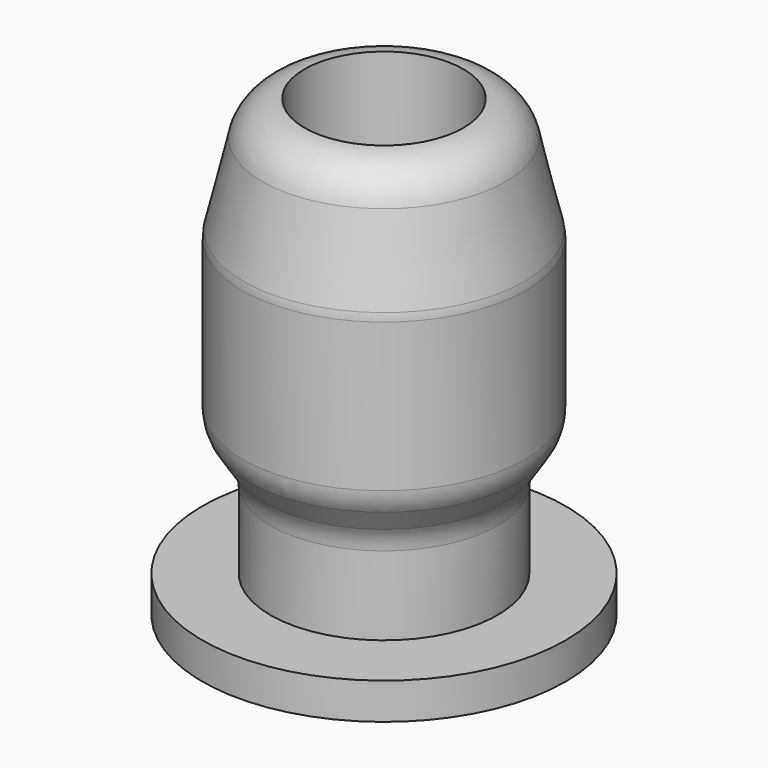
from build123d import *

# Parameters (mm, degrees)
F2_R     = 1.75
F3_DEPTH = 25


# Not quite as in the source:
# - a fillet or chamfer that OpenCascade refuses, or shapes differently, is made with other operations: its cross-section is extruded or revolved along the edge and cut away or added


with BuildPart() as f1:
    # F0 (on Front) → F1 (revolve)
    with BuildSketch(Plane.XZ):
        Polygon((-4, 0), (0, 0), (0, 10), (-2.5, 10), (-3.1176584307, 7.3764383901), (-3.1176584307, 3.7520567627), (-2.5, 2.8), (-2.5, 0.8), (-4, 0.8), align=None)
    revolve(axis=Axis((0, 0, 5), (0, 0, 1)))

    # F2 (on face) → F3 (cut)
    with BuildSketch(Plane.XY.offset(10)):
        Circle(F2_R)
    extrude(amount=-F3_DEPTH, mode=Mode.SUBTRACT)

    # F4: fillet of radius 1 on 7 edges, made by hand

    # F4_s1 → F4_t2 (revolve)
    with BuildSketch(Plane.XZ):
        with BuildLine():
            ThreePointArc((-2.4996, 2.5034415217), (-2.5408144836, 2.7879202783), (-2.6610688008, 3.0490058884))
            Line((-2.6610688008, 3.0490058884), (-2.5769756809, 3.1035623251))
            ThreePointArc((-2.5769756809, 3.1035623251), (-2.4966090641, 2.9789505293), (-2.4159068801, 2.8545564367))
            Line((-2.4159068801, 2.8545564367), (-2.39976, 2.8))
            ThreePointArc((-2.39976, 2.8), (-2.39976, 2.6517207608), (-2.39936, 2.5034415217))
            Line((-2.39936, 2.5034415217), (-2.4996, 2.5034415217))
        make_face()
    revolve(axis=Axis((0, 0, 2.8), (0, 0, 1)))

    # F4_s3 → F4_t4 (revolve, cut)
    with BuildSketch(Plane.XZ):
        with BuildLine():
            ThreePointArc((-1.7069387157, 10.0004), (-2.3289092353, 9.7839522663), (-2.6821291124, 9.2281351497))
            Line((-2.6821291124, 9.2281351497), (-2.7796481521, 9.251093809))
            ThreePointArc((-2.7796481521, 9.251093809), (-2.6883889182, 9.6369804016), (-2.5975190397, 10.0229586592))
            Line((-2.5975190397, 10.0229586592), (-2.5, 10.1001851443))
            ThreePointArc((-2.5, 10.1001851443), (-2.1034693578, 10.1001851443), (-1.7069387157, 10.1005851443))
            Line((-1.7069387157, 10.1005851443), (-1.7069387157, 10.0004))
        make_face()
    revolve(axis=Axis((0, 0, 10), (0, 0, 1)), mode=Mode.SUBTRACT)

    # F4_s5 → F4_t6 (revolve, cut)
    with BuildSketch(Plane.XZ):
        with BuildLine():
            ThreePointArc((-3.0913827866, 7.489792119), (-3.1113671869, 7.3757078111), (-3.1180584307, 7.2600798179))
            Line((-3.1180584307, 7.2600798179), (-3.2182984307, 7.2600798179))
            ThreePointArc((-3.2182984307, 7.2600798179), (-3.2178984307, 7.318259104), (-3.2178984307, 7.3764383901))
            Line((-3.2178984307, 7.3764383901), (-3.2152308663, 7.3994096202))
            ThreePointArc((-3.2152308663, 7.3994096202), (-3.2018983666, 7.4560406522), (-3.1889552222, 7.5127633491))
            Line((-3.1889552222, 7.5127633491), (-3.0913827866, 7.489792119))
        make_face()
    revolve(axis=Axis((0, 0, 7.3764383901), (0, 0, 1)), mode=Mode.SUBTRACT)

    # F4_s7 → F4_t8 (revolve, cut)
    with BuildSketch(Plane.XZ):
        with BuildLine():
            ThreePointArc((-3.1180584307, 4.048615241), (-3.0768439472, 3.7641364844), (-2.9565896299, 3.5030508742))
            Line((-2.9565896299, 3.5030508742), (-3.0406827498, 3.4484944376))
            ThreePointArc((-3.0406827498, 3.4484944376), (-3.1210493667, 3.5731062334), (-3.2017515506, 3.697500326))
            Line((-3.2017515506, 3.697500326), (-3.2178984307, 3.7520567627))
            ThreePointArc((-3.2178984307, 3.7520567627), (-3.2178984307, 3.9003360018), (-3.2182984307, 4.048615241))
            Line((-3.2182984307, 4.048615241), (-3.1180584307, 4.048615241))
        make_face()
    revolve(axis=Axis((0, 0, 3.7520567627), (0, 0, 1)), mode=Mode.SUBTRACT)


solid = f1.part
